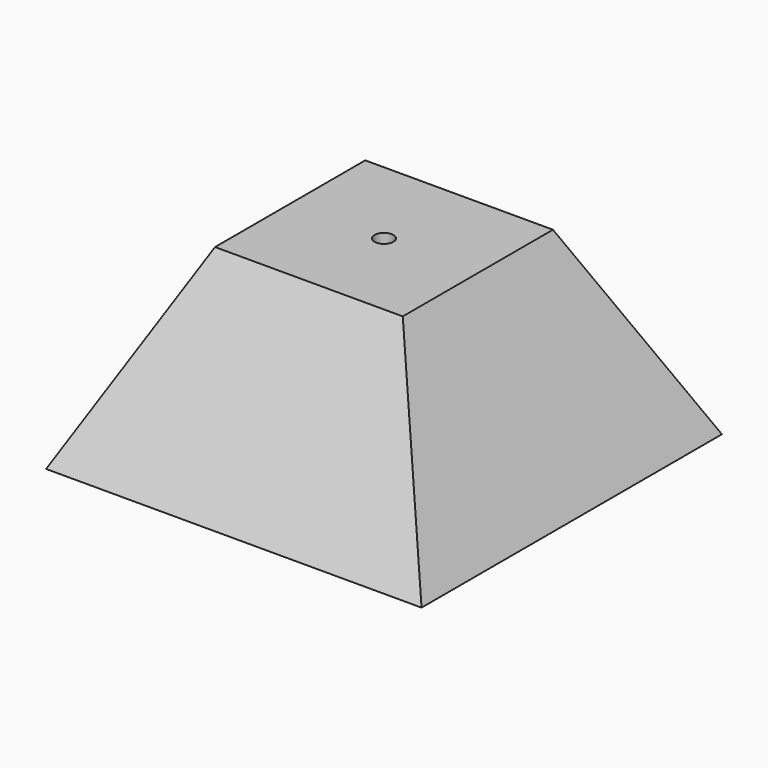
from build123d import *

# Parameters (mm, degrees)
F0_W  = 76.2
F0_H  = 76.2
F2_W  = 38.1
F2_H  = 38.1
F4_W  = 38.1
F4_H  = 38.1
F8_D  = 3.81
F10_D = 3.81


with BuildPart() as f3:
    # F0 (on Top) → F3 section 0
    with BuildSketch(Plane.XY):
        Rectangle(F0_W, F0_H)
    # F2 (on offset) → F3 section 1
    with BuildSketch(Plane.XY.offset(38.1)):
        Rectangle(F2_W, F2_H)
    loft()

    # F10 (through all)
    with Locations(Plane.XY.offset(38.1)):
        with Locations((0, 0)):
            Hole(F10_D / 2)


with BuildPart() as f6:
    # F4 (on offset) → F6 section 0
    with BuildSketch(Plane.XY.offset(38.1), mode=Mode.PRIVATE) as f6_s0:
        Rectangle(F4_W, F4_H)
    loft([f6_s0.sketch, Vertex(0, 0, 76.5771791339)])

    # F8 (through all)
    with Locations(Plane(origin=(0, 0, 38.1), x_dir=(1, 0, 0), z_dir=(0, 0, -1))):
        with Locations((0, 0)):
            Hole(F8_D / 2)


solid = f3.part
